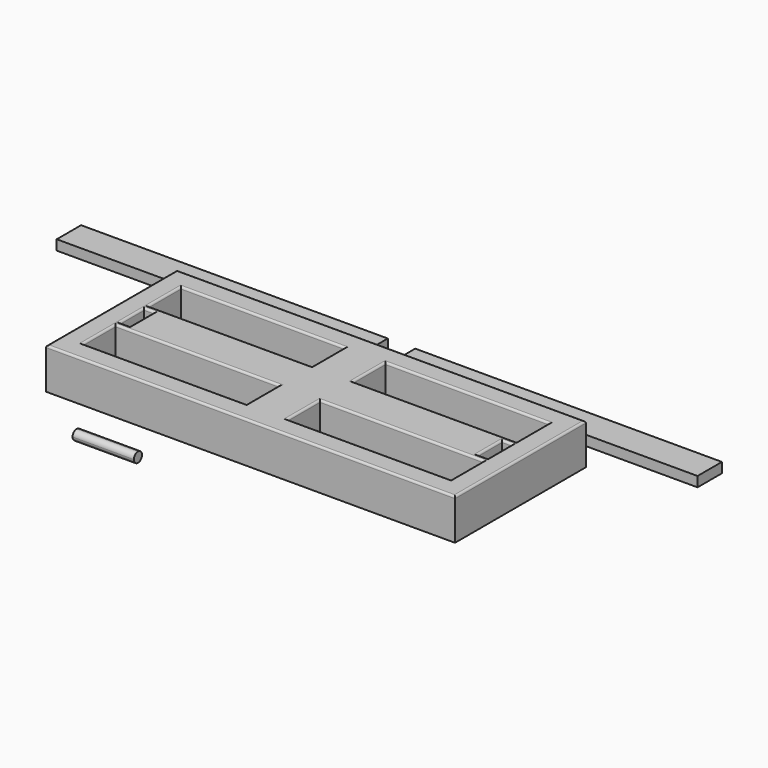
from build123d import *

# Parameters (mm, degrees)
F0_W        = 10
F0_H        = 10
F1_DEPTH    = 20
F0_W_2      = 80
F0_H_2      = 20
F2_DEPTH    = 5
F3_DEPTH    = 5
F4_DEPTH    = 5
F5_DEPTH    = 5
F6_W        = 150
F6_H        = 14.9
F7_DEPTH    = 4.9
F6_W_2      = 30
F6_H_2      = 5
F8_R        = 1
F9_T1_DEPTH = 42.5


# Not quite as in the source:
# - a fillet or chamfer that OpenCascade refuses, or shapes differently, is made with other operations: its cross-section is extruded or revolved along the edge and cut away or added


with BuildPart() as f1:
    # F0 (on Top) → F1 (new body)
    with BuildSketch(Plane.XY):
        Polygon((10, 10), (10, 30), (-10, 30), (-10, 10), (-90, 10), (-90, 7.5), (-85, 7.5), (-85, -7.5), (-90, -7.5), (-90, -10), (-10, -10), (-10, -30), (10, -30), (10, -10), (90, -10), (90, -7.5), (85, -7.5), (85, 7.5), (90, 7.5), (90, 10), align=None)
        Polygon((-90, 10), (-90, 30), (-100, 30), (-100, -30), (-90, -30), (-90, -10), (-90, -7.5), (-90, 7.5), align=None)
        with Locations((-95, -35)):
            Rectangle(F0_W, F0_H)
        Polygon((90, -40), (90, -30), (10, -30), (-10, -30), (-90, -30), (-90, -40), align=None)
        with Locations((-95, 35)):
            Rectangle(F0_W, F0_H)
        Polygon((90, 30), (90, 40), (-90, 40), (-90, 30), (-10, 30), (10, 30), align=None)
        with Locations((95, 35)):
            Rectangle(F0_W, F0_H)
        Polygon((100, -30), (100, 30), (90, 30), (90, 10), (90, 7.5), (90, -7.5), (90, -10), (90, -30), align=None)
        with Locations((95, -35)):
            Rectangle(F0_W, F0_H)
    extrude(amount=F1_DEPTH)

    # F0 (on Top) → F2 (join)
    with BuildSketch(Plane.XY):
        with Locations((-50, 20)):
            Rectangle(F0_W_2, F0_H_2)
    extrude(amount=F2_DEPTH)

    # F0 (on Top) → F3 (join)
    with BuildSketch(Plane.XY):
        with Locations((-50, -20)):
            Rectangle(F0_W_2, F0_H_2)
    extrude(amount=F3_DEPTH)

    # F0 (on Top) → F4 (join)
    with BuildSketch(Plane.XY):
        with Locations((50, 20)):
            Rectangle(F0_W_2, F0_H_2)
    extrude(amount=F4_DEPTH)

    # F0 (on Top) → F5 (join)
    with BuildSketch(Plane.XY):
        with Locations((50, -20)):
            Rectangle(F0_W_2, F0_H_2)
    extrude(amount=F5_DEPTH)

    # F8
    f8_edges = [f1.edges().sort_by_distance(p)[0] for p in [
        (-90, 0, 20),
        (-85, 0, 20),
        (-87.5, 7.5, 20),
        (-87.5, -7.5, 20),
        (85, 0, 20),
        (87.5, 7.5, 20),
        (90, 0, 20),
        (87.5, -7.5, 20),
        (-50, -10, 20),
        (-90, -20, 20),
        (-50, -30, 20),
        (50, -30, 20),
        (-10, -20, 20),
        (50, -10, 20),
        (10, -20, 20),
        (90, -20, 20),
        (0, -40, 20),
        (100, 0, 20),
        (0, 40, 20),
        (-100, 0, 20),
        (-10, 20, 20),
        (-50, 10, 20),
        (-90, 20, 20),
        (-50, 30, 20),
        (10, 20, 20),
        (50, 30, 20),
        (90, 20, 20),
        (50, 10, 20),
    ]]
    fillet(f8_edges, radius=F8_R)


with BuildPart() as f7:
    # F6 (on Top) → F7 (new body)
    with BuildSketch(Plane.XY):
        with Locations((-94.7340503335, 61.1213589191)):
            Rectangle(F6_W, F6_H)
    extrude(amount=F7_DEPTH)


with BuildPart() as f7b:
    # F6 (on Top) → F7, piece 2 (new body)
    with BuildSketch(Plane.XY):
        with Locations((68.6728258617, 61.1213589191)):
            Rectangle(F6_W, F6_H)
    extrude(amount=F7_DEPTH)


with BuildPart() as f7c:
    # F6 (on Top) → F7, piece 3 (new body)
    with BuildSketch(Plane.XY):
        with Locations((-50.844014287, -64.0248632431)):
            Rectangle(F6_W_2, F6_H_2)
    extrude(amount=F7_DEPTH)

    # F9: fillet of radius 2.5 on 4 edges, made by hand

    # F9_s2 → F9_t1 (cut)
    with BuildSketch(Plane.YZ.offset(-72.094014287)):
        with BuildLine():
            ThreePointArc((-66.5248632431, 2.4), (-65.7926301961, 4.167766953), (-64.0248632431, 4.9))
            Line((-64.0248632431, 4.9), (-66.5248632431, 4.9))
            Line((-66.5248632431, 4.9), (-66.5248632431, 2.4))
        make_face()
        with BuildLine():
            ThreePointArc((-61.5248632431, 2.4), (-62.2570962901, 4.167766953), (-64.0248632431, 4.9))
            Line((-64.0248632431, 4.9), (-61.5248632431, 4.9))
            Line((-61.5248632431, 4.9), (-61.5248632431, 2.4))
        make_face()
        with BuildLine():
            ThreePointArc((-66.5248632431, 2.5), (-65.7926301961, 0.732233047), (-64.0248632431, 0))
            Line((-64.0248632431, 0), (-66.5248632431, 0))
            Line((-66.5248632431, 0), (-66.5248632431, 2.5))
        make_face()
        with BuildLine():
            ThreePointArc((-61.5248632431, 2.5), (-62.2570962901, 0.732233047), (-64.0248632431, 0))
            Line((-64.0248632431, 0), (-61.5248632431, 0))
            Line((-61.5248632431, 0), (-61.5248632431, 2.5))
        make_face()
    extrude(amount=F9_T1_DEPTH, mode=Mode.SUBTRACT)


solid = Compound([f1.part, f7.part, f7b.part, f7c.part])
